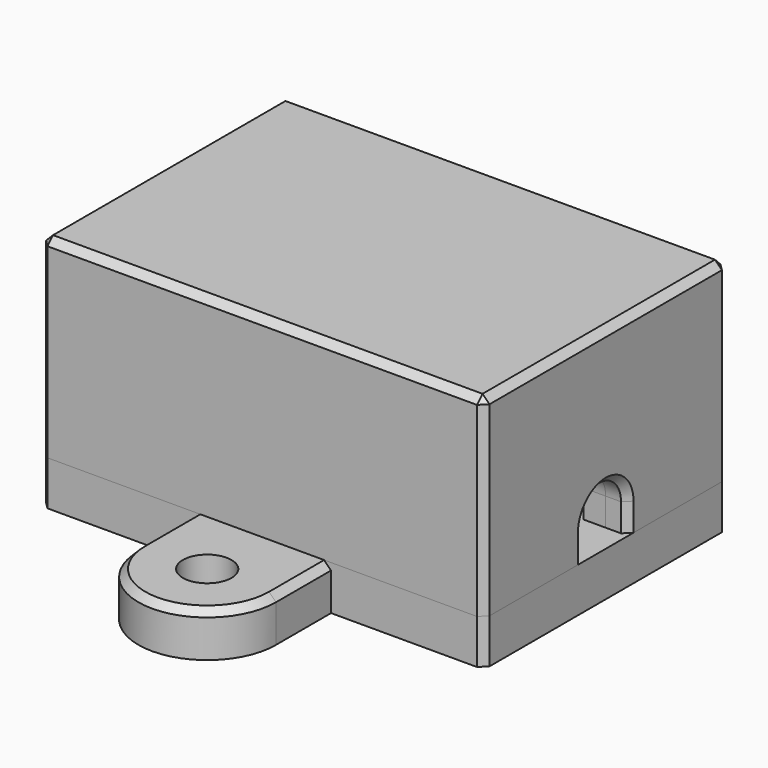
from build123d import *

# Parameters (mm, degrees)
F2_W       = 2
F2_H       = 15.5
F2_W_2     = 13.5
F2_W_3     = 1.6
F2_H_2     = 14
F2_W_4     = 4
F2_R       = 1.75
F3_DEPTH   = 3.2
F4_DEPTH   = 3.2
F5_DEPTH   = 4.5
F6_DEPTH   = 10.7
F7_DEPTH   = 10.7
F8_START   = 10.7
F8_DEPTH   = 3.2
F10_DEPTH  = 3.2
F11_SIZE   = 0.5
F11_2_SIZE = 0.5


with BuildPart() as f3:
    # F2 (on Top) → F3 (new body)
    with BuildSketch(Plane.XY):
        Polygon((7.2, 3.2), (3.2, 3.2), (3.2, 3.95), (1.6, 3.95), (1.6, 1.6), (30.3, 1.6), (30.3, 20.3), (1.6, 20.3), (1.6, 17.95), (3.2, 17.95), (3.2, 18.7), (7.2, 18.7), (9.2, 18.7), (22.7, 18.7), (24.7, 18.7), (28.7, 18.7), (28.7, 3.2), (24.7, 3.2), (22.7, 3.2), (9.2, 3.2), align=None)
        Polygon((3.2, 3.95), (3.2, 3.2), (7.2, 3.2), (7.2, 18.7), (3.2, 18.7), (3.2, 17.95), align=None)
        with Locations((23.7, 10.95)):
            Rectangle(F2_W, F2_H)
        with Locations((15.95, 10.95)):
            Rectangle(F2_W_2, F2_H)
        with Locations((2.4, 10.95)):
            Rectangle(F2_W_3, F2_H_2)
        with Locations((0.8, 10.95)):
            Rectangle(F2_W_3, F2_H_2)
        with Locations((26.7, 10.95)):
            Rectangle(F2_W_4, F2_H)
        with Locations((8.2, 10.95)):
            Rectangle(F2_W, F2_H)
        Polygon((1.6, 1.6), (1.6, 3.95), (0, 3.95), (0, 0), (11, 0), (20.9, 0), (31.9, 0), (31.9, 21.9), (20.9, 21.9), (11, 21.9), (0, 21.9), (0, 17.95), (1.6, 17.95), (1.6, 20.3), (30.3, 20.3), (30.3, 1.6), align=None)
        with BuildLine():
            Line((11, 26.85), (11, 21.9))
            Line((11, 21.9), (20.9, 21.9))
            Line((20.9, 21.9), (20.9, 26.85))
            ThreePointArc((20.9, 26.85), (15.95, 31.8), (11, 26.85))
        make_face()
        with Locations((15.95, 26.85)):
            Circle(F2_R, mode=Mode.SUBTRACT)
        with BuildLine():
            Line((20.9, 0), (11, 0))
            Line((11, 0), (11, -4.95))
            ThreePointArc((11, -4.95), (15.95, -9.9), (20.9, -4.95))
            Line((20.9, -4.95), (20.9, 0))
        make_face()
        with Locations((15.95, -4.95)):
            Circle(F2_R, mode=Mode.SUBTRACT)
    extrude(amount=-F3_DEPTH)

    # F2 (on Top) → F4 (join)
    with BuildSketch(Plane.XY):
        with Locations((8.2, 10.95)):
            Rectangle(F2_W, F2_H)
        with Locations((23.7, 10.95)):
            Rectangle(F2_W, F2_H)
    extrude(amount=F4_DEPTH)

    # F2 (on Top) → F5 (join)
    with BuildSketch(Plane.XY):
        with Locations((0.8, 10.95)):
            Rectangle(F2_W_3, F2_H_2)
        with Locations((2.4, 10.95)):
            Rectangle(F2_W_3, F2_H_2)
    extrude(amount=F5_DEPTH)

    # F2 (on Top) → F6 (join)
    with BuildSketch(Plane.XY):
        Polygon((7.2, 3.2), (3.2, 3.2), (3.2, 3.95), (1.6, 3.95), (1.6, 1.6), (30.3, 1.6), (30.3, 20.3), (1.6, 20.3), (1.6, 17.95), (3.2, 17.95), (3.2, 18.7), (7.2, 18.7), (9.2, 18.7), (22.7, 18.7), (24.7, 18.7), (28.7, 18.7), (28.7, 3.2), (24.7, 3.2), (22.7, 3.2), (9.2, 3.2), align=None)
    extrude(amount=F6_DEPTH)


with BuildPart() as f7:
    # F2 (on Top) → F7 (new body)
    with BuildSketch(Plane.XY):
        Polygon((1.6, 1.6), (1.6, 3.95), (0, 3.95), (0, 0), (11, 0), (20.9, 0), (31.9, 0), (31.9, 21.9), (20.9, 21.9), (11, 21.9), (0, 21.9), (0, 17.95), (1.6, 17.95), (1.6, 20.3), (30.3, 20.3), (30.3, 1.6), align=None)
    extrude(amount=F7_DEPTH)

    # F2 (on Top) → F8 (join)
    with BuildSketch(Plane.XY.offset(F8_START)):
        with Locations((0.8, 10.95)):
            Rectangle(F2_W_3, F2_H_2)
        Polygon((1.6, 1.6), (1.6, 3.95), (0, 3.95), (0, 0), (11, 0), (20.9, 0), (31.9, 0), (31.9, 21.9), (20.9, 21.9), (11, 21.9), (0, 21.9), (0, 17.95), (1.6, 17.95), (1.6, 20.3), (30.3, 20.3), (30.3, 1.6), align=None)
        with Locations((8.2, 10.95)):
            Rectangle(F2_W, F2_H)
        with Locations((15.95, 10.95)):
            Rectangle(F2_W_2, F2_H)
        with Locations((23.7, 10.95)):
            Rectangle(F2_W, F2_H)
        Polygon((7.2, 3.2), (3.2, 3.2), (3.2, 3.95), (1.6, 3.95), (1.6, 1.6), (30.3, 1.6), (30.3, 20.3), (1.6, 20.3), (1.6, 17.95), (3.2, 17.95), (3.2, 18.7), (7.2, 18.7), (9.2, 18.7), (22.7, 18.7), (24.7, 18.7), (28.7, 18.7), (28.7, 3.2), (24.7, 3.2), (22.7, 3.2), (9.2, 3.2), align=None)
        with Locations((26.7, 10.95)):
            Rectangle(F2_W_4, F2_H)
        Polygon((3.2, 3.95), (3.2, 3.2), (7.2, 3.2), (7.2, 18.7), (3.2, 18.7), (3.2, 17.95), align=None)
        with Locations((2.4, 10.95)):
            Rectangle(F2_W_3, F2_H_2)
    extrude(amount=F8_DEPTH)


with BuildPart() as f10_tool:
    # F9 (on face) → F10 (new body, through all)
    with BuildSketch(Plane.YZ.offset(31.9)):
        with BuildLine():
            Line((12.95, 0), (12.95, 2))
            ThreePointArc((12.95, 2), (10.95, 4), (8.95, 2))
            Line((8.95, 2), (8.95, 0))
            Line((8.95, 0), (12.95, 0))
        make_face()
    extrude(amount=-F10_DEPTH)


with BuildPart() as f3_1:
    add(f3.part)

    # F10: cut by f10_tool
    add(f10_tool.part, mode=Mode.SUBTRACT)

    # F11
    f11_edges = [f3_1.edges().sort_by_distance(p)[0] for p in [
        (0, 21.9, -1.6),
        (0, 0, -1.6),
        (31.9, 0, -1.6),
        (31.9, 21.9, -1.6),
        (15.95, 31.8, 0),
        (15.95, -9.9, 0),
        (11, 24.375, 0),
        (20.9, 24.375, 0),
        (20.9, -2.475, 0),
        (11, -2.475, 0),
    ]]
    chamfer(f11_edges, length=F11_SIZE)


with BuildPart() as f7_1:
    add(f7.part)

    # F10: cut by f10_tool
    add(f10_tool.part, mode=Mode.SUBTRACT)

    # F11#2
    f11_2_edges = [f7_1.edges().sort_by_distance(p)[0] for p in [
        (15.95, 0, 13.9),
        (31.9, 10.95, 13.9),
        (15.95, 21.9, 13.9),
        (0, 10.95, 13.9),
        (0, 21.9, 6.95),
        (0, 0, 6.95),
        (31.9, 0, 6.95),
        (31.9, 21.9, 6.95),
        (31.9, 12.95, 1),
        (31.9, 8.95, 1),
        (31.9, 10.95, 4),
    ]]
    chamfer(f11_2_edges, length=F11_2_SIZE)


solid = Compound([f3_1.part, f7_1.part])
